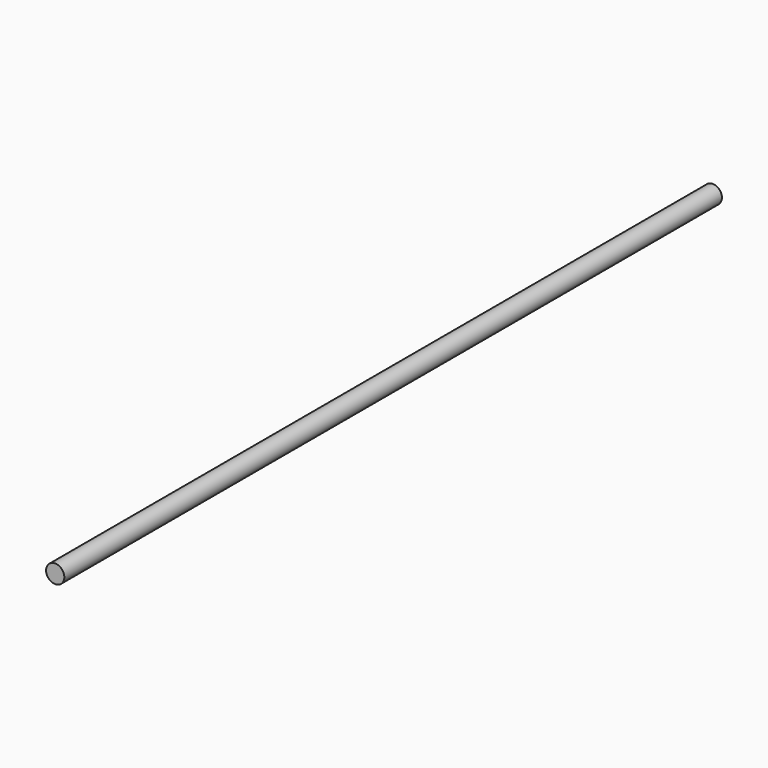
from build123d import *

# Parameters (mm, degrees)
F0_R     = 6.35
F1_DEPTH = 469.9


# Not quite as in the source:
# - a pattern or mirror of a feature is missing from the dataset's text; its kind, count and spacing are read off the source's solid


with BuildPart() as f1:
    # F0 (on Front) → F1 (new body)
    with BuildSketch(Plane.XZ):
        Circle(F0_R)
    extrude(amount=F1_DEPTH)

    # F1_copies: F1 across plane


with BuildPart() as f1_1:
    add(f1.part)
    add(f1.part.mirror(Plane(origin=(0, -285.75, 0), x_dir=(0, 0, -1), z_dir=(0, -1, 0))))


solid = f1_1.part
